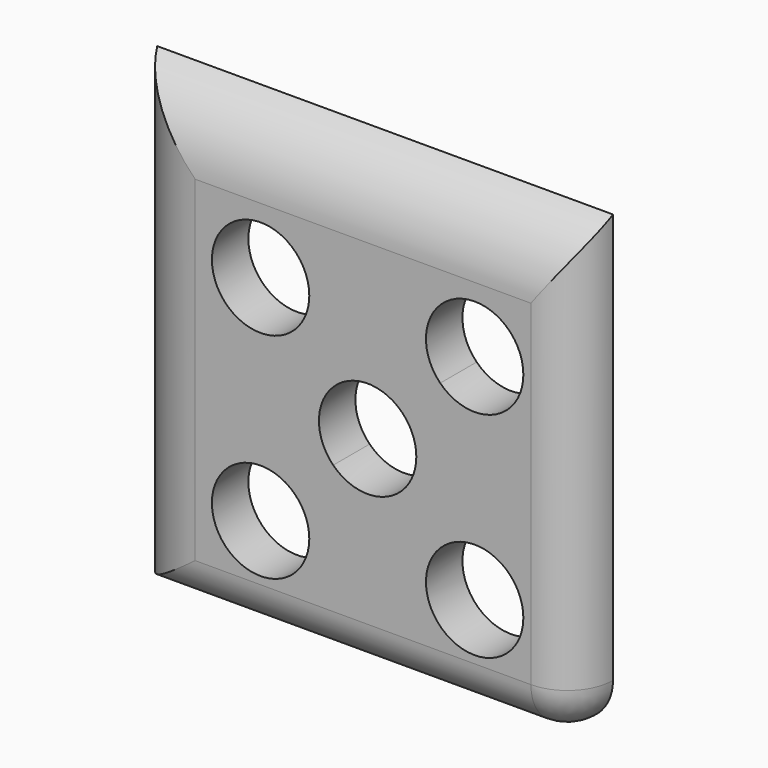
from build123d import *

# Parameters (mm, degrees)
F0_W        = 21.5
F0_H        = 21.5
F0_W_2      = 5.5
F0_H_2      = 5.5
F0_W_3      = 3
F0_H_3      = 3
F1_DEPTH    = 3
F2_R        = 2.99999
F3_T1_DEPTH = 51.4949074278
F4_T1_DEPTH = 46.5959279422


# Not quite as in the source:
# - a fillet or chamfer that OpenCascade refuses, or shapes differently, is made with other operations: its cross-section is extruded or revolved along the edge and cut away or added
# - a fillet or chamfer is up to 0.001 mm smaller than in the source, because OpenCascade refuses the exact size


with BuildPart() as f1:
    # F0 (on Front) → F1 (new body)
    with BuildSketch(Plane.XZ):
        with Locations((16.25, 13.75)):
            Rectangle(F0_W, F0_H)
        with BuildLine():
            ThreePointArc((11.4712772337, 8.9712772337), (12.1660339017, 7.9315004007), (12.41, 6.705))
            ThreePointArc((12.41, 6.705), (6.2439660983, 5.4784995993), (11.4712772337, 8.9712772337))
        make_face(mode=Mode.SUBTRACT)
        with BuildLine():
            ThreePointArc((26.5, 6.705), (22.0684995993, 3.7439660983), (21.0287227663, 8.9712772337))
            ThreePointArc((21.0287227663, 8.9712772337), (24.5215004007, 9.6660339017), (26.5, 6.705))
        make_face(mode=Mode.SUBTRACT)
        with BuildLine():
            ThreePointArc((18.5162772337, 11.4837227663), (16.25, 10.545), (13.9837227663, 11.4837227663))
            ThreePointArc((13.9837227663, 11.4837227663), (13.045, 13.75), (13.9837227663, 16.0162772337))
            ThreePointArc((13.9837227663, 16.0162772337), (16.25, 16.955), (18.5162772337, 16.0162772337))
            ThreePointArc((18.5162772337, 16.0162772337), (19.2110339017, 14.9765004007), (19.455, 13.75))
            ThreePointArc((19.455, 13.75), (19.2110339017, 12.5234995993), (18.5162772337, 11.4837227663))
        make_face(mode=Mode.SUBTRACT)
        with BuildLine():
            ThreePointArc((12.41, 20.795), (12.1660339017, 19.5684995993), (11.4712772337, 18.5287227663))
            ThreePointArc((11.4712772337, 18.5287227663), (6.2439660983, 22.0215004007), (12.41, 20.795))
        make_face(mode=Mode.SUBTRACT)
        with BuildLine():
            ThreePointArc((26.5, 20.795), (24.5215004007, 17.8339660983), (21.0287227663, 18.5287227663))
            ThreePointArc((21.0287227663, 18.5287227663), (22.0684995993, 23.7560339017), (26.5, 20.795))
        make_face(mode=Mode.SUBTRACT)
        with Locations((2.75, 13.75)):
            Rectangle(F0_W_2, F0_H)
        with Locations((2.75, 27.25)):
            Rectangle(F0_W_2, F0_H_2)
        with Locations((16.25, 27.25)):
            Rectangle(F0_W, F0_H_2)
        with Locations((28.5, 27.25)):
            Rectangle(F0_W_3, F0_H_2)
        with Locations((28.5, 13.75)):
            Rectangle(F0_W_3, F0_H)
        with BuildLine():
            Line((27, 3), (27, 0))
            ThreePointArc((27, 0), (29.1213203436, 0.8786796564), (30, 3))
            Line((30, 3), (27, 3))
        make_face()
        with Locations((16.25, 1.5)):
            Rectangle(F0_W, F0_H_3)
        with Locations((2.75, 1.5)):
            Rectangle(F0_W_2, F0_H_3)
    extrude(amount=F1_DEPTH)

    # F2 (radius 3 in the source; OpenCascade refuses exactly that, so slightly less here)
    f2_edges = [f1.edges().sort_by_distance(p)[0] for p in [
        (29.12132, -3, 0.87868),
        (13.5, -3, 0),
        (30, -3, 16.5),
    ]]
    fillet(f2_edges, radius=F2_R)

    # F3: fillet of radius 5.5 on 1 edges, made by hand

    # F3_s2 → F3_t1 (cut)
    with BuildSketch(Plane.XY.offset(-9.2474587139)):
        with BuildLine():
            ThreePointArc((4.8989794856, -3), (2.0266981623, -2.1904157598), (0, 0))
            Line((0, 0), (0, -3))
            Line((0, -3), (4.8989794856, -3))
        make_face()
    extrude(amount=F3_T1_DEPTH, mode=Mode.SUBTRACT)

    # F4: fillet of radius 5.5 on 1 edges, made by hand

    # F4_s2 → F4_t1 (cut)
    with BuildSketch(Plane.YZ.offset(-7.3484692283)):
        with BuildLine():
            ThreePointArc((0, 30), (-2.1904157598, 27.9733018377), (-3, 25.1010205144))
            Line((-3, 25.1010205144), (-3, 30))
            Line((-3, 30), (0, 30))
        make_face()
    extrude(amount=F4_T1_DEPTH, mode=Mode.SUBTRACT)


solid = f1.part
